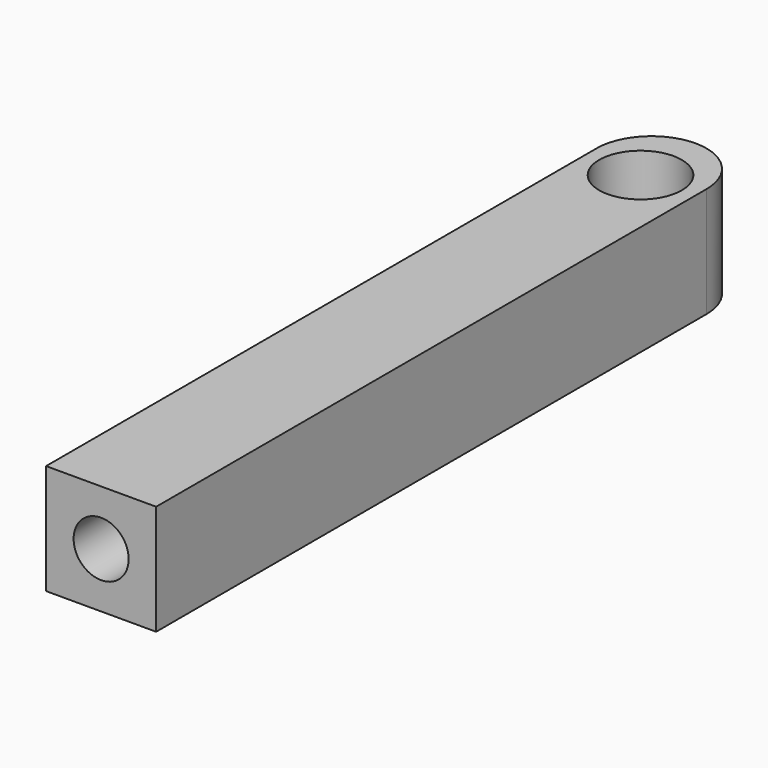
from build123d import *

# Parameters (mm, degrees)
F0_W     = 25.4
F0_H     = 171.45
F0_R     = 9.525
F1_DEPTH = 25.4
F2_R     = 12.69999
F3_R     = 6.35
F4_DEPTH = 25.4


# Not quite as in the source:
# - a fillet or chamfer is up to 0.001 mm smaller than in the source, because OpenCascade refuses the exact size


with BuildPart() as f1:
    # F0 (on Top) → F1 (new body)
    with BuildSketch(Plane.XY):
        with Locations((-33.2050182253, -27.8180489531)):
            Rectangle(F0_W, F0_H)
        with Locations((-33.2050182253, 42.0319510469)):
            Circle(F0_R, mode=Mode.SUBTRACT)
    extrude(amount=-F1_DEPTH)

    # F2 (radius 12.7 in the source; OpenCascade refuses exactly that, so slightly less here)
    f2_edges = [f1.edges().sort_by_distance(p)[0] for p in [
        (-45.905018, 57.906951, -12.7),
        (-20.505018, 57.906951, -12.7),
    ]]
    fillet(f2_edges, radius=F2_R)

    # F3 (on face) → F4 (cut)
    with BuildSketch(Plane.XZ.offset(113.5430489531)):
        with Locations((-33.2050182253, -12.7)):
            Circle(F3_R)
    extrude(amount=-F4_DEPTH, mode=Mode.SUBTRACT)


solid = f1.part
